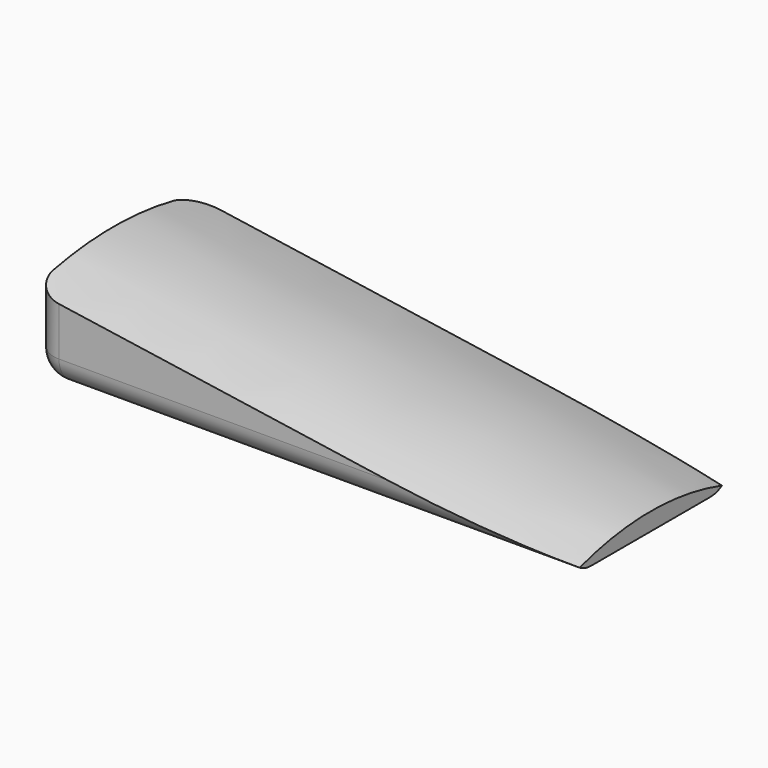
from build123d import *

# Parameters (mm, degrees)
F4_DEPTH               = 101.6
DRAFT_F4_DRAFTED_ANGLE = -8
F6_DEPTH               = 101.601
F7_W                   = 34.925
F7_H                   = 38.1
F8_DEPTH               = 101.601
F9_R                   = 5.08


# Not quite as in the source:
# - an extrude with a draft is written as a straight extrude whose walls are then drafted


with BuildPart() as f4:
    # F0 (on Right) → F4 (new body)
    with BuildSketch(Plane.YZ):
        with BuildLine():
            Line((-47.4402376048, 30.48), (47.4402376048, 30.48))
            ThreePointArc((47.4402376048, 30.48), (0, 56.388), (-47.4402376048, 30.48))
        make_face()
    extrude(amount=-F4_DEPTH)

    # draft_F4_drafted
    draft_f4_drafted_walls = [f4.faces().sort_by_distance(p)[0] for p in [
        (-67.7333333333, 0, 30.48),
        (-67.7333333333, 0, 56.388),
    ]]
    draft(draft_f4_drafted_walls, neutral_plane=Plane(origin=(0, 0, 0), x_dir=(0, 1, 0), z_dir=(-1, 0, 0)), angle=DRAFT_F4_DRAFTED_ANGLE)

    # F5 (on face) → F6 (cut, through all)
    with BuildSketch(Plane(origin=(-101.6, 0, 0), x_dir=(0, -1, 0), z_dir=(-1, 0, 0))):
        with BuildLine():
            ThreePointArc((68.7847628019, 16.2010511942), (60.6109524283, 36.333594637), (46.7068010332, 53.0310511942))
            Line((46.7068010332, 53.0310511942), (-46.7068010332, 53.0310511942))
            ThreePointArc((-46.7068010332, 53.0310511942), (-60.6109524283, 36.333594637), (-68.7847628019, 16.2010511942))
            Line((-68.7847628019, 16.2010511942), (68.7847628019, 16.2010511942))
        make_face()
    extrude(amount=-F6_DEPTH, mode=Mode.SUBTRACT)

    # F7 (on face) → F8 (cut, through all)
    with BuildSketch(Plane.YZ):
        with Locations((-36.6279416394, 72.0810511942)):
            Rectangle(F7_W, F7_H)
        with Locations((36.6279416394, 72.0810511942)):
            Rectangle(F7_W, F7_H)
    extrude(amount=-F8_DEPTH, mode=Mode.SUBTRACT)

    # F9
    f9_edges = [f4.edges().sort_by_distance(p)[0] for p in [
        (-101.6, -19.165442, 60.524728),
        (-101.6, 19.165442, 60.524728),
        (-50.8, 19.165442, 53.031051),
        (-50.8, -19.165442, 53.031051),
        (-101.6, 0, 53.031051),
    ]]
    fillet(f9_edges, radius=F9_R)


solid = f4.part
